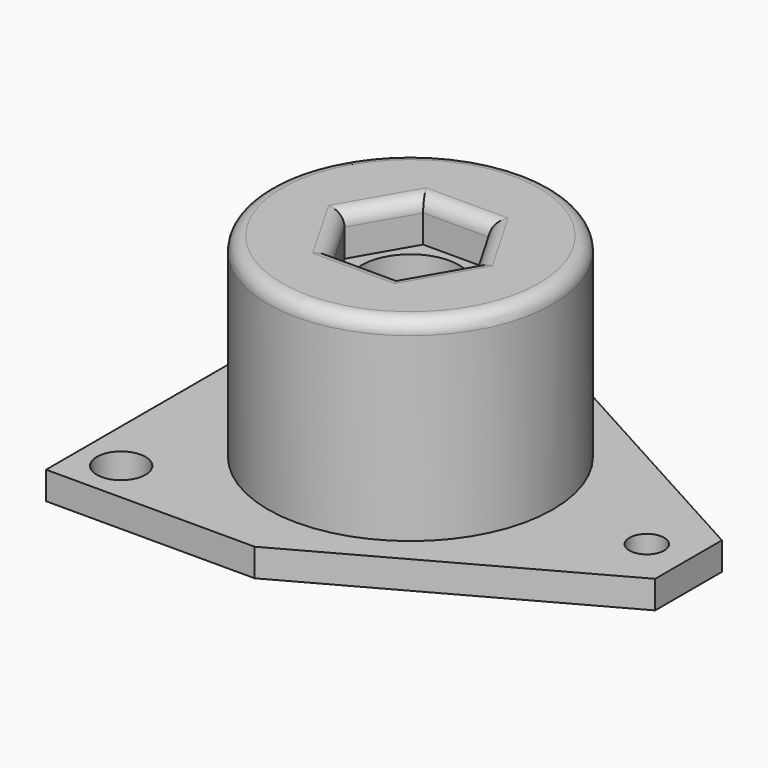
from build123d import *

# Parameters (mm, degrees)
F0_R     = 1.25
F0_R_2   = 1.75
F1_DEPTH = 2
F2_R     = 10.25
F2_R_2   = 3.5
F3_DEPTH = 14
F4_R     = 3.5
F5_DEPTH = 3
F6_R     = 1


with BuildPart() as f1:
    # F0 (on Top) → F1 (new body)
    with BuildSketch(Plane.XY):
        with BuildLine():
            ThreePointArc((0, 3.5), (2.474874, 2.474874), (3.5, 0))
            ThreePointArc((3.5, 0), (2.474874, -2.474874), (0, -3.5))
            Line((0, -3.5), (0, -14))
            Line((0, -14), (20, -3))
            Line((20, -3), (20, 0))
            Line((20, 0), (20, 3))
            Line((20, 3), (0, 14))
            Line((0, 14), (0, 3.5))
        make_face()
        with Locations((17, 0)):
            Circle(F0_R, mode=Mode.SUBTRACT)
        with BuildLine():
            ThreePointArc((0, -3.5), (-3.5, 0), (0, 3.5))
            Line((0, 3.5), (0, 14))
            Line((0, 14), (-15, 14))
            Line((-15, 14), (-15, -14))
            Line((-15, -14), (0, -14))
            Line((0, -14), (0, -3.5))
        make_face()
        with Locations((-12, -11)):
            Circle(F0_R_2, mode=Mode.SUBTRACT)
        with Locations((-12, 11)):
            Circle(F0_R_2, mode=Mode.SUBTRACT)
    extrude(amount=F1_DEPTH)

    # F2 (on face) → F3 (join)
    with BuildSketch(Plane.XY.offset(2)):
        Circle(F2_R)
        Circle(F2_R_2, mode=Mode.SUBTRACT)
    extrude(amount=F3_DEPTH)

    # F4 (on face) → F5 (cut)
    with BuildSketch(Plane.XY.offset(16)):
        Polygon((-2.367136, -4.1), (2.367136, -4.1), (4.734272, 0), (2.367136, 4.1), (-2.367136, 4.1), (-4.734272, 0), align=None)
        Circle(F4_R, mode=Mode.SUBTRACT)
    extrude(amount=-F5_DEPTH, mode=Mode.SUBTRACT)

    # F6
    f6_edges = [f1.edges().sort_by_distance(p)[0] for p in [
        (-3.550704, 2.05, 16),
        (0, 4.1, 16),
        (3.550704, 2.05, 16),
        (3.550704, -2.05, 16),
        (0, -4.1, 16),
        (-3.550704, -2.05, 16),
        (-10.25, 0, 16),
    ]]
    fillet(f6_edges, radius=F6_R)


solid = f1.part
